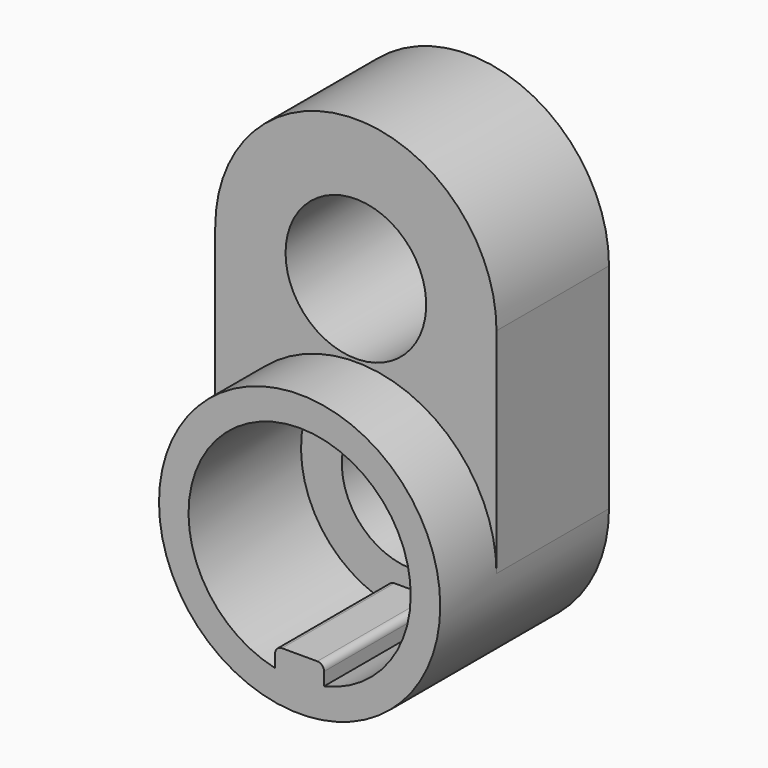
from build123d import *

# Parameters (mm, degrees)
F0_R     = 6.35
F0_R_2   = 3.175
F1_DEPTH = 3.175
F2_R     = 6.35
F2_R_2   = 5.0165
F3_DEPTH = 6.35
F4_R     = 3.175
F5_DEPTH = 6.35
F7_DEPTH = 6.35
F8_R     = 0.3048


# Not quite as in the source:
# - a feature names something its author has since deleted; it is built from what else it names


with BuildPart() as f1:
    # F0 (on Front) → F1 (new body)
    with BuildSketch(Plane.XZ):
        Circle(F0_R)
        Circle(F0_R_2, mode=Mode.SUBTRACT)
    extrude(amount=F1_DEPTH)

    # F2 (on face) → F3 (join)
    with BuildSketch(Plane.XZ.offset(3.175)):
        Circle(F2_R)
        Circle(F2_R_2, mode=Mode.SUBTRACT)
    extrude(amount=F3_DEPTH)

    # F4 (on face) → F5 (join)
    with BuildSketch(Plane(origin=(0, 0, 0), x_dir=(-1, 0, 0), z_dir=(0, 1, 0))):
        with BuildLine():
            ThreePointArc((-6.35, 9.652), (-5.7675394704, 6.9953125029), (-4.1270115096, 4.826))
            ThreePointArc((-4.1270115096, 4.826), (0, 6.35), (4.1270115096, 4.826))
            ThreePointArc((4.1270115096, 4.826), (5.7675394704, 6.9953125029), (6.35, 9.652))
            ThreePointArc((6.35, 9.652), (0, 16.002), (-6.35, 9.652))
        make_face()
        with Locations((0, 9.652)):
            Circle(F4_R, mode=Mode.SUBTRACT)
        with BuildLine():
            Line((-6.35, 9.652), (-6.35, 0))
            ThreePointArc((-6.35, 0), (-5.7675394704, 2.6566874971), (-4.1270115096, 4.826))
            ThreePointArc((-4.1270115096, 4.826), (-5.7675394704, 6.9953125029), (-6.35, 9.652))
        make_face()
        with BuildLine():
            ThreePointArc((4.1270115096, 4.826), (5.7675394704, 2.6566874971), (6.35, 0))
            Line((6.35, 0), (6.35, 9.652))
            ThreePointArc((6.35, 9.652), (5.7675394704, 6.9953125029), (4.1270115096, 4.826))
        make_face()
    extrude(amount=-F5_DEPTH)

    # F6 (on face) → F7 (join, through all)
    with BuildSketch(Plane.XZ.offset(9.525)):
        with BuildLine():
            Line((-1.1049, -4.0005), (-1.1049, -4.8933085167))
            ThreePointArc((-1.1049, -4.8933085167), (0, -5.0165), (1.1049, -4.8933085167))
            Line((1.1049, -4.8933085167), (1.1049, -4.0005))
            Line((1.1049, -4.0005), (-1.1049, -4.0005))
        make_face()
    extrude(amount=-F7_DEPTH)

    # F8
    f8_edges = [f1.edges().sort_by_distance(p)[0] for p in [
        (1.1049, -6.35, -4.0005),
        (-1.1049, -6.35, -4.0005),
    ]]
    fillet(f8_edges, radius=F8_R)


solid = f1.part
